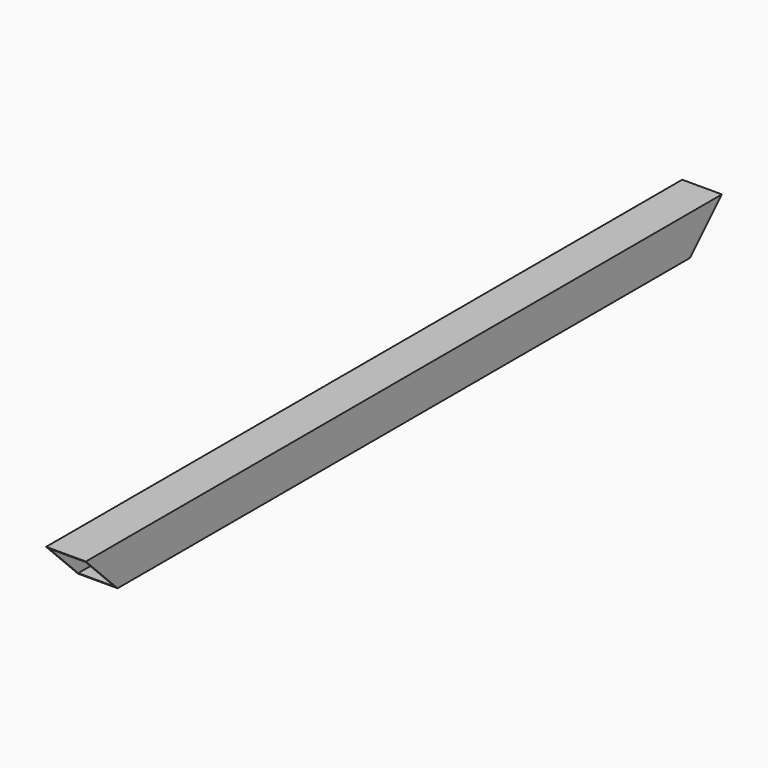
from build123d import *

# Parameters (mm, degrees)
F0_W     = 50
F0_H     = 50
F0_W_2   = 46
F0_H_2   = 46
F1_DEPTH = 1000
F3_DEPTH = 50.001


# Not quite as in the source:
# - a pattern or mirror of a feature is missing from the dataset's text; its kind, count and spacing are read off the source's solid


with BuildPart() as f1:
    # F0 (on Front) → F1 (new body)
    with BuildSketch(Plane.XZ):
        with Locations((25, 25)):
            Rectangle(F0_W, F0_H)
        with Locations((25, 25)):
            Rectangle(F0_W_2, F0_H_2, mode=Mode.SUBTRACT)
    extrude(amount=F1_DEPTH)

    # F2 (on face) → F3 (cut, through all)
    with BuildSketch(Plane.YZ.offset(50)):
        Polygon((-950, 0), (-1000, 50), (-1000, 0), align=None)
    f3 = extrude(amount=-F3_DEPTH, mode=Mode.SUBTRACT)

    # F3_copies: F3 across plane
    add(f3.mirror(Plane.ZX.offset(-500)), mode=Mode.SUBTRACT)


solid = f1.part
